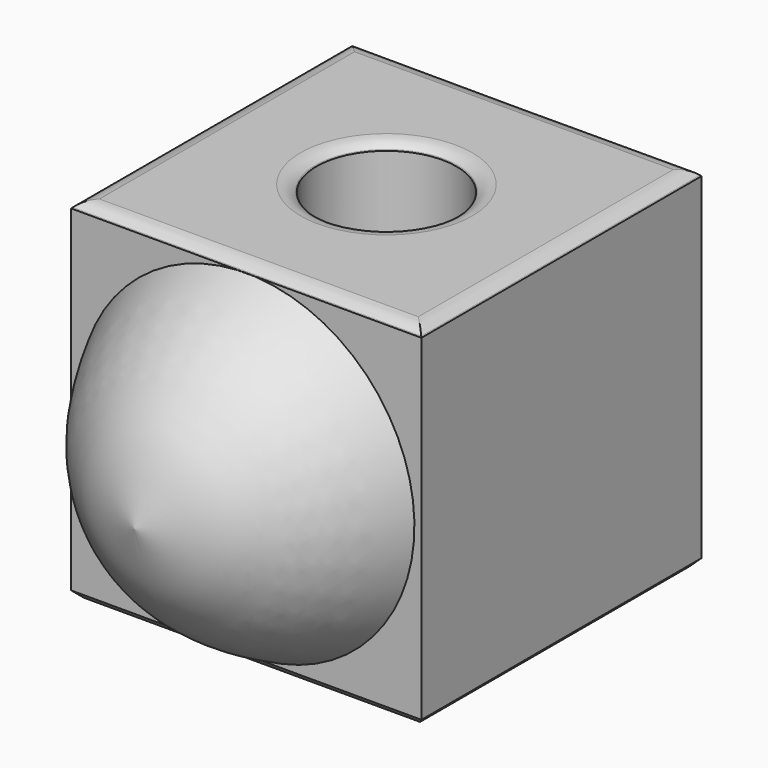
from build123d import *

# Parameters (mm, degrees)
F0_W        = 50
F0_H        = 50
F1_DEPTH    = 50
F2_R        = 10
F1_FACE_W   = 50
F1_FACE_H   = 50
F3_DEPTH    = 50.001
F4_SIZE     = 1
F5_T1_DEPTH = 54.2132034356
F5_T3_DEPTH = 54.2132034356


# Not quite as in the source:
# - a fillet or chamfer that OpenCascade refuses, or shapes differently, is made with other operations: its cross-section is extruded or revolved along the edge and cut away or added


with BuildPart() as f1:
    # F0 (on Top) → F1 (new body)
    with BuildSketch(Plane.XY):
        Rectangle(F0_W, F0_H)
    extrude(amount=F1_DEPTH)

    # F2 (on Top) + F1_face (on face) → F3 (cut, through all)
    with BuildSketch(Plane.XY):
        Circle(F2_R)
    with BuildSketch(Plane.XY.offset(50)):
        Rectangle(F1_FACE_W, F1_FACE_H)
    extrude(amount=F3_DEPTH, mode=Mode.SUBTRACT)

    # F4
    f4_edges = [f1.edges().sort_by_distance(p)[0] for p in [
        (25, 0, 0),
        (0, -25, 0),
        (0, 25, 0),
        (-25, 0, 0),
        (-10, 0, 0),
        (25, 0, 50),
        (0, -25, 50),
        (0, 25, 50),
        (-25, 0, 50),
        (-10, 0, 50),
    ]]
    chamfer(f4_edges, length=F4_SIZE)

    # F5: fillet of radius 3 on 5 edges, made by hand

    # F5_s2 → F5_t1 (cut)
    with BuildSketch(Plane.XZ.offset(-27.1066017178)):
        with BuildLine():
            add(Edge.make_bspline(
                [(24.8786796564, 49.1213203436), (24, 50), (22.7573593129, 50)],
                knots=[0, 0, 0, 1, 1, 1], degree=2, weights=[1, 1, 1]))
            Line((22.7573593129, 50), (24, 50))
            Line((24, 50), (24.8786796564, 49.1213203436))
        make_face()
        with BuildLine():
            add(Edge.make_bspline(
                [(-22.7573593129, 50), (-24, 50), (-24.8786796564, 49.1213203436)],
                knots=[0, 0, 0, 1, 1, 1], degree=2, weights=[1, 1, 1]))
            Line((-24.8786796564, 49.1213203436), (-24, 50))
            Line((-24, 50), (-22.7573593129, 50))
        make_face()
    extrude(amount=F5_T1_DEPTH, mode=Mode.SUBTRACT)

    # F5_s4 → F5_t3 (cut)
    with BuildSketch(Plane.YZ.offset(-27.1066017178)):
        with BuildLine():
            add(Edge.make_bspline(
                [(-24.8786796564, 49.1213203436), (-24, 50), (-22.7573593129, 50)],
                knots=[0, 0, 0, 1, 1, 1], degree=2, weights=[1, 1, 1]))
            Line((-22.7573593129, 50), (-24, 50))
            Line((-24, 50), (-24.8786796564, 49.1213203436))
        make_face()
        with BuildLine():
            add(Edge.make_bspline(
                [(22.7573593129, 50), (24, 50), (24.8786796564, 49.1213203436)],
                knots=[0, 0, 0, 1, 1, 1], degree=2, weights=[1, 1, 1]))
            Line((24.8786796564, 49.1213203436), (24, 50))
            Line((24, 50), (22.7573593129, 50))
        make_face()
    extrude(amount=F5_T3_DEPTH, mode=Mode.SUBTRACT)

    # F5_s5 → F5_t6 (revolve, cut)
    with BuildSketch(Plane.XZ):
        with BuildLine():
            add(Edge.make_bspline(
                [(12.2426406871, 50), (11, 50), (10.1213203436, 49.1213203436)],
                knots=[0, 0, 0, 1, 1, 1], degree=2, weights=[1, 1, 1]))
            Line((10.1213203436, 49.1213203436), (11, 50))
            Line((11, 50), (12.2426406871, 50))
        make_face()
    revolve(axis=Axis((0, 0, 50), (0, 0, -1)), mode=Mode.SUBTRACT)


with BuildPart() as f7:
    # F6 (on Right) → F7 (revolve)
    with BuildSketch(Plane.YZ):
        with BuildLine():
            Line((-25, 1), (-25, 25))
            Line((-25, 25), (-45, 25))
            add(Edge.make_bspline(
                [(-45, 25), (-42.9437309504, 16.5351219475), (-39.3878491982, 12.0366081686), (-33.9029468596, 5.3530973382), (-25, 1)],
                knots=[0, 0, 0, 0, 0.4742530664, 1, 1, 1, 1], degree=3))
        make_face()
    revolve(axis=Axis((0, -35, 25), (0, -1, 0)))


solid = Compound([f1.part, f7.part])
